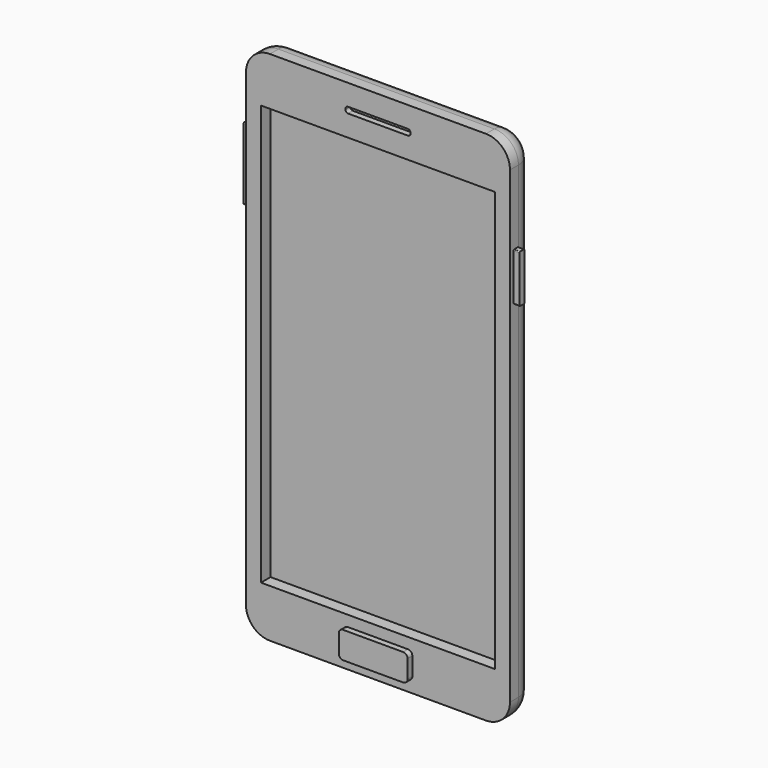
from build123d import *

# Parameters (mm, degrees)
F1_DEPTH  = 7.874
F2_R      = 5.08
F3_W      = 61.9125
F3_H      = 111.125
F4_DEPTH  = 3.175
F6_DEPTH  = 1.5875
F7_DEPTH  = 1.5875
F9_DEPTH  = 1.5875
F11_DEPTH = 1.5875


# Not quite as in the source:
# - a length typed as a fraction of an inch, garbled in the dataset ("3 / 203.2 mm" for 3/8 in), is restored
# - a feature names something its author has since deleted; it is built from what else it names


with BuildPart() as f1:
    # F0 (on Front) → F1 (new body)
    with BuildSketch(Plane.XZ):
        with BuildLine():
            ThreePointArc((-28.575, 68.326), (-33.0651280605, 66.4661280605), (-34.925, 61.976))
            Line((-34.925, 61.976), (-34.925, -61.976))
            ThreePointArc((-34.925, -61.976), (-33.0651280605, -66.4661280605), (-28.575, -68.326))
            Line((-28.575, -68.326), (28.575, -68.326))
            ThreePointArc((28.575, -68.326), (33.0651280605, -66.4661280605), (34.925, -61.976))
            Line((34.925, -61.976), (34.925, 61.976))
            ThreePointArc((34.925, 61.976), (33.0651280605, 66.4661280605), (28.575, 68.326))
            Line((28.575, 68.326), (-28.575, 68.326))
        make_face()
    extrude(amount=F1_DEPTH)

    # F2
    f2_edges = [f1.edges().sort_by_distance(p)[0] for p in [
        (33.065128, 0, 66.466128),
        (0, 0, 68.326),
        (34.925, 0, 0),
    ]]
    fillet(f2_edges, radius=F2_R)

    # F3 (on face) → F4 (cut)
    with BuildSketch(Plane.XZ.offset(7.874)):
        Rectangle(F3_W, F3_H)
    extrude(amount=-F4_DEPTH, mode=Mode.SUBTRACT)

    # F5 (on face) → F6 (join)
    with BuildSketch(Plane.XZ.offset(7.874)):
        with BuildLine():
            Line((7.9375, -58.4327856867), (-7.9375, -58.4327856867))
            ThreePointArc((-7.9375, -58.4327856867), (-8.7591312506, -58.7731164939), (-9.0994620578, -59.5947477445))
            Line((-9.0994620578, -59.5947477445), (-9.0994620578, -64.3572522555))
            ThreePointArc((-9.0994620578, -64.3572522555), (-8.7591311338, -65.1788836228), (-7.9374996698, -65.5192143133))
            Line((-7.9374996698, -65.5192143133), (7.9375003302, -65.5192098023))
            ThreePointArc((7.9375003302, -65.5192098023), (8.7591313673, -65.1788788783), (9.0994620578, -64.3572477445))
            Line((9.0994620578, -64.3572477445), (9.0994620578, -59.5947477445))
            ThreePointArc((9.0994620578, -59.5947477445), (8.7591312506, -58.7731164939), (7.9375, -58.4327856867))
        make_face()
    extrude(amount=F6_DEPTH)

    # F3 (on face) → F7 (cut)
    with BuildSketch(Plane.XZ.offset(7.874)):
        with BuildLine():
            Line((7.9375, 62.76975), (-7.9375, 62.76975))
            ThreePointArc((-7.9375, 62.76975), (-8.4134535744, 62.5726035744), (-8.6106, 62.09665))
            Line((-8.6106, 62.09665), (-8.6106, 61.85535))
            ThreePointArc((-8.6106, 61.85535), (-8.4134535744, 61.3793964256), (-7.9375, 61.18225))
            Line((-7.9375, 61.18225), (7.9375, 61.18225))
            ThreePointArc((7.9375, 61.18225), (8.4134535744, 61.3793964256), (8.6106, 61.85535))
            Line((8.6106, 61.85535), (8.6106, 62.09665))
            ThreePointArc((8.6106, 62.09665), (8.4134535744, 62.5726035744), (7.9375, 62.76975))
        make_face()
    extrude(amount=-F7_DEPTH, mode=Mode.SUBTRACT)

    # F8 (on face) → F9 (join)
    with BuildSketch(Plane(origin=(-34.925, 0, 0), x_dir=(0, -1, 0), z_dir=(-1, 0, 0))):
        with BuildLine():
            Line((6.6675, 30.4519287544), (6.6675, 49.0500712456))
            ThreePointArc((6.6675, 49.0500712456), (6.601327, 49.209827), (6.4415712456, 49.276))
            Line((6.4415712456, 49.276), (5.3059287544, 49.276))
            ThreePointArc((5.3059287544, 49.276), (5.146173, 49.209827), (5.08, 49.0500712456))
            Line((5.08, 49.0500712456), (5.08, 30.4519287544))
            ThreePointArc((5.08, 30.4519287544), (5.146173, 30.292173), (5.3059287544, 30.226))
            Line((5.3059287544, 30.226), (6.4415712456, 30.226))
            ThreePointArc((6.4415712456, 30.226), (6.601327, 30.292173), (6.6675, 30.4519287544))
        make_face()
    extrude(amount=F9_DEPTH)

    # F10 (on face) → F11 (join)
    with BuildSketch(Plane.YZ.offset(34.925)):
        with BuildLine():
            Line((-5.08, 30.4519287544), (-5.08, 42.7000712456))
            ThreePointArc((-5.08, 42.7000712456), (-5.146173, 42.859827), (-5.3059287544, 42.926))
            Line((-5.3059287544, 42.926), (-6.4415712456, 42.926))
            ThreePointArc((-6.4415712456, 42.926), (-6.601327, 42.859827), (-6.6675, 42.7000712456))
            Line((-6.6675, 42.7000712456), (-6.6675, 30.4519287544))
            ThreePointArc((-6.6675, 30.4519287544), (-6.601327, 30.292173), (-6.4415712456, 30.226))
            Line((-6.4415712456, 30.226), (-5.3059287544, 30.226))
            ThreePointArc((-5.3059287544, 30.226), (-5.146173, 30.292173), (-5.08, 30.4519287544))
        make_face()
    extrude(amount=F11_DEPTH)


solid = f1.part
